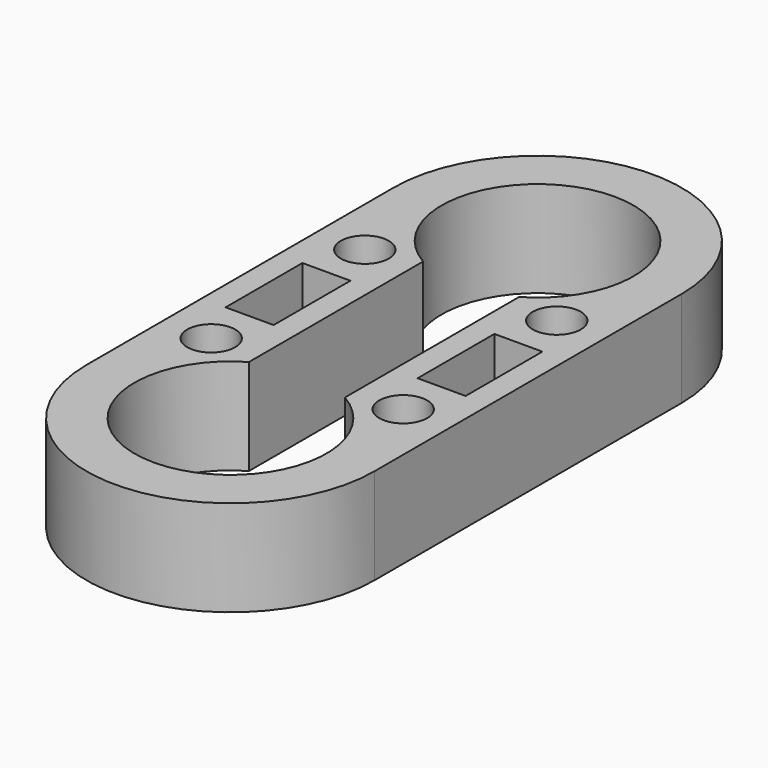
from build123d import *

# Parameters (mm, degrees)
F0_R     = 6.35
F0_W     = 12.7
F0_H     = 25.4
F1_DEPTH = 25.4


# Not quite as in the source:
# - ends of sketch curves that miss each other by under 0.0002 mm in the source are joined


with BuildPart() as f1:
    # F0 (on Top) → F1 (new body)
    with BuildSketch(Plane.XY):
        with BuildLine():
            ThreePointArc((38.1, 50.8), (0, 88.9), (-38.1, 50.8))
            Line((-38.1, 50.8), (-38.1, -50.8))
            ThreePointArc((-38.1, -50.8), (0, -88.9), (38.1, -50.8))
            Line((38.1, -50.8), (38.1, 50.8))
        make_face()
        with Locations((-25.4, -25.4)):
            Circle(F0_R, mode=Mode.SUBTRACT)
        with Locations((25.4, -25.4)):
            Circle(F0_R, mode=Mode.SUBTRACT)
        with Locations((-25.4, 0)):
            Rectangle(F0_W, F0_H, mode=Mode.SUBTRACT)
        with Locations((-25.4, 25.4)):
            Circle(F0_R, mode=Mode.SUBTRACT)
        with BuildLine():
            Line((-12.7, -28.802965), (-12.7, 28.802965))
            ThreePointArc((-12.7, 28.802965), (0, 76.2), (12.700004441, 28.8029573079))
            Line((12.700004441, 28.8029573079), (12.7, -28.802965))
            ThreePointArc((12.7, -28.802965), (0, -76.2), (-12.7, -28.802965))
        make_face(mode=Mode.SUBTRACT)
        with Locations((25.4, 0)):
            Rectangle(F0_W, F0_H, mode=Mode.SUBTRACT)
        with Locations((25.4, 25.4)):
            Circle(F0_R, mode=Mode.SUBTRACT)
    extrude(amount=F1_DEPTH)


solid = f1.part
